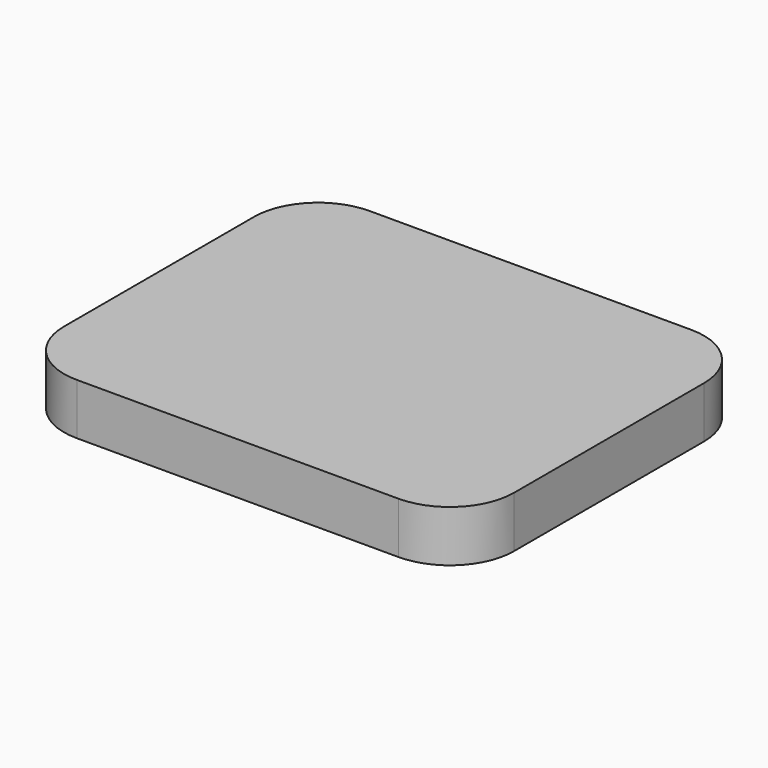
from build123d import *

# Parameters (mm, degrees)
F0_TEXT_SIZE = 11.755370735
F1_DEPTH     = 3
F2_W         = 70.076478878
F2_H         = 56.9664388895
F3_DEPTH     = 8
F4_R         = 10


# Not quite as in the source:
# - Text() gives the source's letters only with a copy of the font that has no kerning and outlines rounded to 1/6400 em; it was checked with that copy


with BuildPart() as f1:
    # F0 (on Top) → F1 (new body)
    with BuildSketch(Plane.XY):
        with Locations((0, 0.0620995217)):
            Text('Handmade', F0_TEXT_SIZE, font='Open Sans', font_style=FontStyle.BOLDITALIC, text_align=(TextAlign.LEFT, TextAlign.BOTTOM))
        with Locations((24.4364769154, -15.9252046779)):
            Text('By', F0_TEXT_SIZE, font='Open Sans', font_style=FontStyle.BOLDITALIC, text_align=(TextAlign.LEFT, TextAlign.BOTTOM))
        with Locations((0, -31.9125088775)):
            Text('Tim Garner', F0_TEXT_SIZE, font='Open Sans', font_style=FontStyle.BOLDITALIC, text_align=(TextAlign.LEFT, TextAlign.BOTTOM))
    extrude(amount=F1_DEPTH)


with BuildPart() as f3:
    # F2 (on face) → F3 (new body)
    with BuildSketch(Plane.XY.offset(3)):
        with Locations((31.2033974333, -11.2350471318)):
            Rectangle(F2_W, F2_H)
        Polygon((3.2768095924, -31.9125088775), (1.5263614189, -31.9125088775), (2.9847621007, -25.0007182407), (0.9643077556, -25.0007182407), (1.2802333441, -23.5202762387), (7.0771005378, -23.5202762387), (6.7611749493, -25.0007182407), (4.7352102742, -25.0007182407), align=None, mode=Mode.SUBTRACT)
        Polygon((2.9847621007, -25.0007182407), (1.5263614189, -31.9125088775), (3.2768095924, -31.9125088775), (4.7352102742, -25.0007182407), (6.7611749493, -25.0007182407), (7.0771005378, -23.5202762387), (1.2802333441, -23.5202762387), (0.9643077556, -25.0007182407), align=None)
    extrude(amount=F3_DEPTH)

    # F4
    f4_edges = [f3.edges().sort_by_distance(p)[0] for p in [
        (-3.834842, -39.718267, 7),
        (-3.834842, 17.248172, 7),
        (66.241637, 17.248172, 7),
        (66.241637, -39.718267, 7),
    ]]
    fillet(f4_edges, radius=F4_R)


solid = Compound([f1.part, f3.part])
